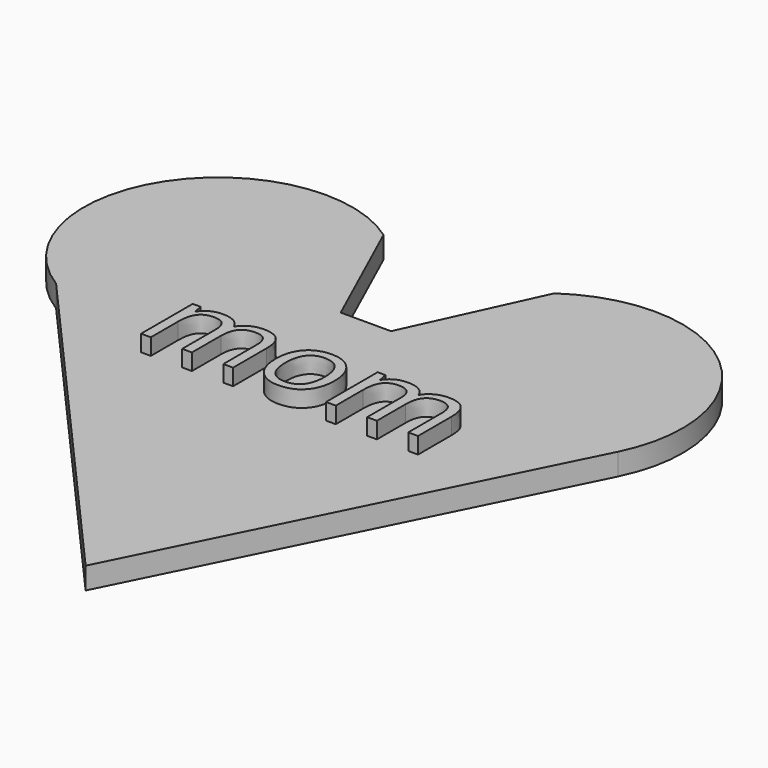
from build123d import *

# Parameters (mm, degrees)
F1_DEPTH     = 2
F2_TEXT_SIZE = 11.0276741907
F3_DEPTH     = 1.5


# Not quite as in the source:
# - Text() gives the source's letters only with a copy of the font that has no kerning and outlines rounded to 1/6400 em; it was checked with that copy


with BuildPart() as f1:
    # F0 (on Top) → F1 (new body)
    with BuildSketch(Plane.XY):
        with BuildLine():
            Line((-22.4454262335, 41.9500422796), (-27.5670554484, 53.2470435135))
            ThreePointArc((-27.5670554484, 53.2470435135), (-44.9232527726, 49.9973415134), (-41.1213325642, 32.7536890181))
            Line((-41.1213325642, 32.7536890181), (-12.2170461524, 0))
            Line((-12.2170461524, 0), (6.4596237368, 37.5129549651))
            ThreePointArc((6.4596237368, 37.5129549651), (3.3538801014, 52.9752732581), (-12.3957438048, 53.7988492039))
            Line((-12.3957438048, 53.7988492039), (-17.8447769581, 41.9500422796))
            Line((-17.8447769581, 41.9500422796), (-22.4454262335, 41.9500422796))
        make_face()
    extrude(amount=F1_DEPTH)

    # F2 (on face) → F3 (join)
    with BuildSketch(Plane.XY.offset(2)):
        with Locations((-30.6908600032, 28.2478053123)):
            Text('mom', F2_TEXT_SIZE, font='Open Sans', text_align=(TextAlign.LEFT, TextAlign.BOTTOM))
    extrude(amount=F3_DEPTH)


solid = f1.part
